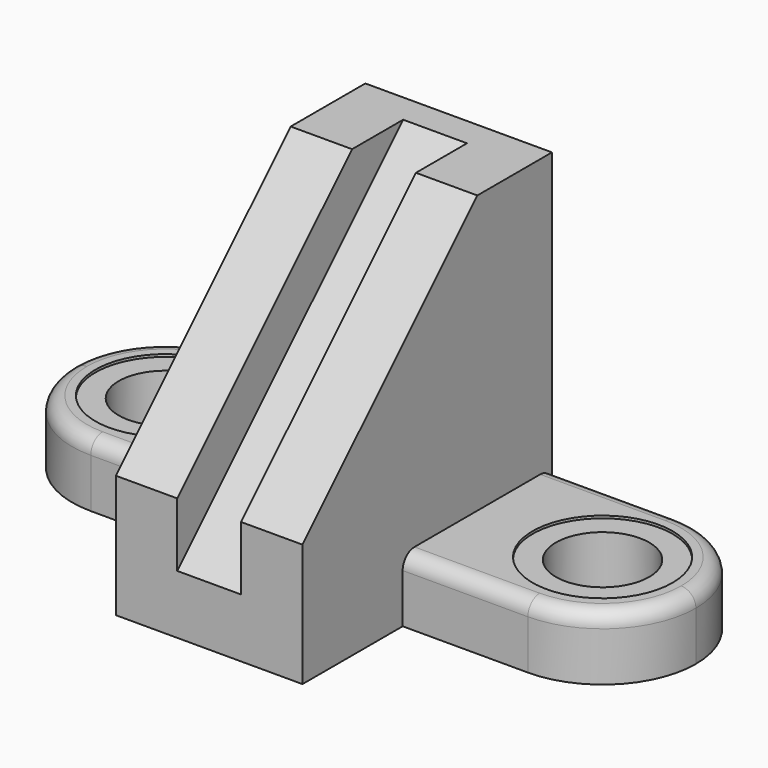
from build123d import *

# Parameters (mm, degrees)
F0_W      = 127
F0_H      = 139
F1_DEPTH  = 76
F3_W      = 76
F3_H      = 26
F4_DEPTH  = 51
F2_W      = 76
F2_H      = 26
F5_DEPTH  = 51
F6_DEPTH  = 38
F7_DEPTH  = 38
F8_R      = 19
F9_DEPTH  = 26.001
F10_R     = 37.99999
F11_R     = 28.5
F11_R_2   = 19
F13_DEPTH = 1
F12_R     = 28.5
F12_R_2   = 19
F14_DEPTH = 1
F15_R     = 6
F17_DEPTH = 165.001
F18_W     = 26
F18_H     = 125.8650070512
F21_DEPTH = 18.3847763109
F22_DEPTH = 26.8710576851
F23_DEPTH = 35.3563390593


# Not quite as in the source:
# - a fillet or chamfer is up to 0.001 mm smaller than in the source, because OpenCascade refuses the exact size


with BuildPart() as f1:
    # F0 (on Right) → F1 (new body)
    with BuildSketch(Plane.YZ):
        with Locations((-63.5, -69.5)):
            Rectangle(F0_W, F0_H)
    extrude(amount=F1_DEPTH)

    # F3 (on face) → F4 (join)
    with BuildSketch(Plane.YZ.offset(76)):
        with Locations((-38, -126)):
            Rectangle(F3_W, F3_H)
    extrude(amount=F4_DEPTH)

    # F2 (on face) → F5 (join)
    with BuildSketch(Plane(origin=(0, 0, 0), x_dir=(0, -1, 0), z_dir=(-1, 0, 0))):
        with Locations((38, -126)):
            Rectangle(F2_W, F2_H)
    extrude(amount=F5_DEPTH)

    # F6 (add): a face of the model
    f6_faces = [f1.faces().sort_by_distance(p)[0] for p in [
        (-51, -38, -126),
    ]]
    extrude(f6_faces, amount=F6_DEPTH)

    # F7 (add): a face of the model
    f7_faces = [f1.faces().sort_by_distance(p)[0] for p in [
        (127, -38, -126),
    ]]
    extrude(f7_faces, amount=F7_DEPTH)

    # F8 (on face) → F9 (cut, through all)
    with BuildSketch(Plane.XY.offset(-113)):
        with Locations((-51, -38)):
            Circle(F8_R)
        with Locations((127, -38)):
            Circle(F8_R)
    extrude(amount=-F9_DEPTH, mode=Mode.SUBTRACT)

    # F10 (radius 38 in the source; OpenCascade refuses exactly that, so slightly less here)
    f10_edges = [f1.edges().sort_by_distance(p)[0] for p in [
        (-89, 0, -126),
        (-89, -76, -126),
        (165, -76, -126),
        (165, 0, -126),
    ]]
    fillet(f10_edges, radius=F10_R)

    # F11 (on face) → F13 (cut)
    with BuildSketch(Plane.XY.offset(-113)):
        with Locations((-51, -38)):
            Circle(F11_R)
        with Locations((-51, -38)):
            Circle(F11_R_2, mode=Mode.SUBTRACT)
    extrude(amount=-F13_DEPTH, mode=Mode.SUBTRACT)

    # F12 (on face) → F14 (cut)
    with BuildSketch(Plane.XY.offset(-113)):
        with Locations((127, -38)):
            Circle(F12_R)
        with Locations((127, -38)):
            Circle(F12_R_2, mode=Mode.SUBTRACT)
    extrude(amount=-F14_DEPTH, mode=Mode.SUBTRACT)

    # F15
    f15_edges = [f1.edges().sort_by_distance(p)[0] for p in [
        (-25.500005, -76, -113),
        (-77.870061, -11.129939, -113),
        (101.500005, -76, -113),
    ]]
    fillet(f15_edges, radius=F15_R)

    # F16 (on face) → F17 (cut, through all)
    with BuildSketch(Plane(origin=(0, 0, 0), x_dir=(0, -1, 0), z_dir=(-1, 0, 0))):
        Polygon((127, 0), (38, 0), (127, -89), align=None)
    extrude(amount=-F17_DEPTH, mode=Mode.SUBTRACT)

    # F18 (on face) → F21 (cut, through all)
    with BuildSketch(Plane(origin=(0, -19, 19), x_dir=(1, 0, 0), z_dir=(0, -0.7071067812, 0.7071067812))):
        with Locations((38, -89.8025612107)):
            Rectangle(F18_W, F18_H)
    extrude(amount=-F21_DEPTH, mode=Mode.SUBTRACT)

    # F22 (cut, through all): a face of the model
    f22_faces = [f1.faces().sort_by_distance(p)[0] for p in [
        (38, -31.5, -6.5),
    ]]
    extrude(f22_faces, amount=-F22_DEPTH, mode=Mode.SUBTRACT)

    # F23 (cut, through all): a face of the model
    f23_faces = [f1.faces().sort_by_distance(p)[0] for p in [
        (38, -120.5, -95.5),
    ]]
    extrude(f23_faces, amount=-F23_DEPTH, mode=Mode.SUBTRACT)


solid = f1.part
